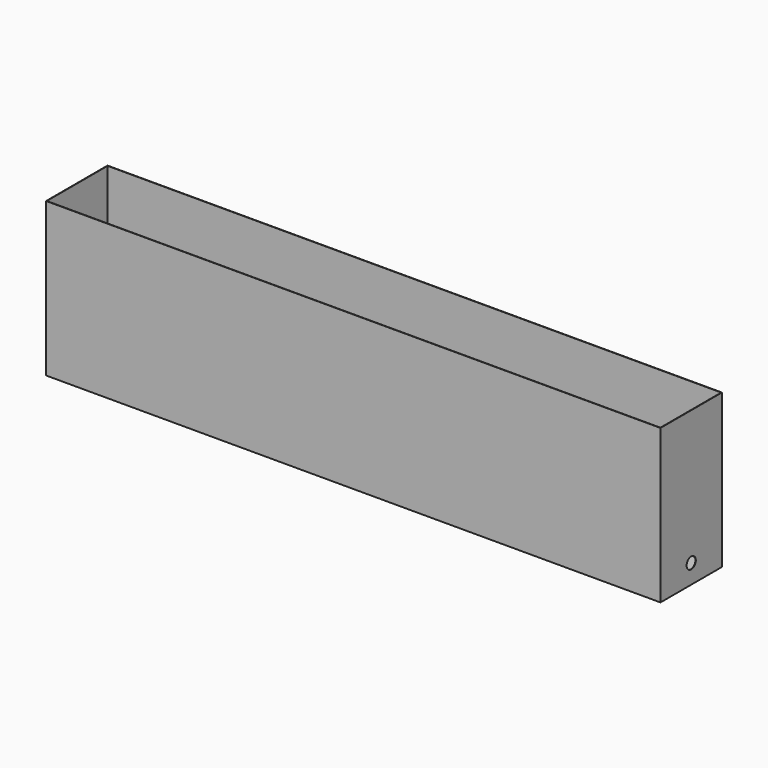
from build123d import *

# Parameters (mm, degrees)
F0_W     = 1600
F0_H     = 200
F1_DEPTH = 400
F2_T     = -1
F5_D     = 40
F8_D     = 30


# Not quite as in the source:
# - the program builds the solid bodies; features that only make, move or delete a surface that nothing else refers to are left out


with BuildPart() as f1:
    # F0 (on Top) → F1 (new body)
    with BuildSketch(Plane.XY):
        Rectangle(F0_W, F0_H)
    extrude(amount=F1_DEPTH)

    # F2
    f2_openings = [f1.faces().sort_by_distance(p)[0] for p in [
        (0, 0, 400),
    ]]
    offset(amount=F2_T, openings=f2_openings)

    # F5 (through all)
    with Locations(Plane.XY.offset(1)):
        with Locations((777, 77), (777, -77), (-777, 77), (-777, -77)):
            Hole(F5_D / 2)

    # F8 (through all)
    with Locations(Plane(origin=(-800, 0, 0), x_dir=(0, -1, 0), z_dir=(-1, 0, 0))):
        with Locations((0, 50)):
            Hole(F8_D / 2)


solid = f1.part
